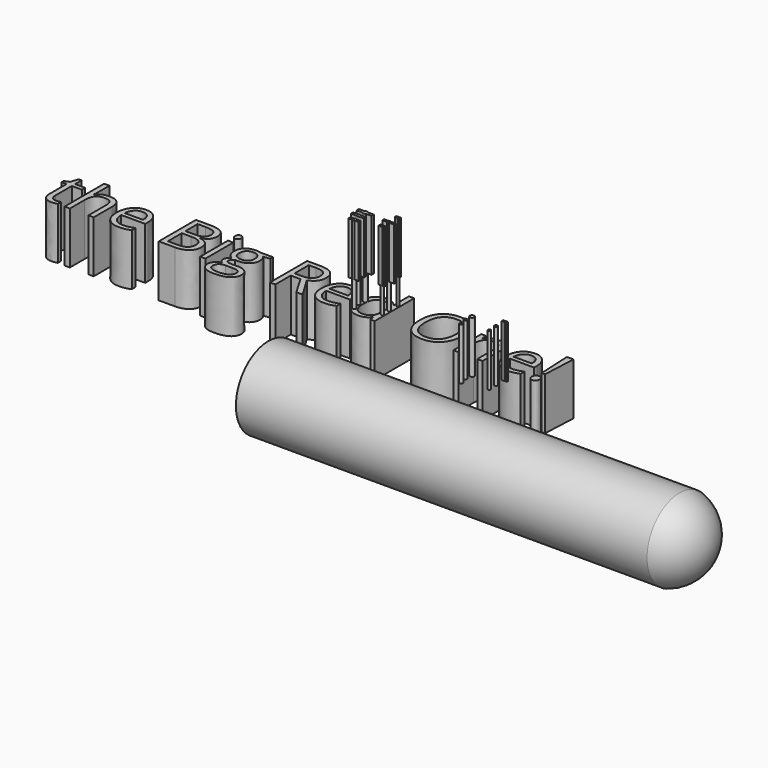
from build123d import *

# Parameters (mm, degrees)
F2_TEXT_SIZE = 31.8179838359
F3_DEPTH     = 25.4
F4_R         = 1.1140946011
F4_R_2       = 0.7578695581
F4_R_3       = 0.853310294
F4_R_4       = 0.5642153701
F4_R_5       = 0.7545312037
F4_R_6       = 0.6707809487
F5_DEPTH     = 12.7
F7_DEPTH     = 25.4
F6_R         = 0.853310294
F6_R_2       = 0.7578695581
F6_R_3       = 1.1140946011
F6_R_4       = 0.6707809487
F6_R_5       = 0.7545312037


# Not quite as in the source:
# - Text() gives the source's letters only with a copy of the font that has no kerning and outlines rounded to 1/6400 em; it was checked with that copy


with BuildPart() as f1:
    # F0 (on Top) → F1 (revolve)
    with BuildSketch(Plane.XY):
        with BuildLine():
            Line((-109.392100472, 19.84375), (-109.392100472, 0))
            Line((-109.392100472, 0), (86.664149528, 0))
            Line((86.664149528, 0), (106.507899528, 0))
            ThreePointArc((106.507899528, 0), (102.3549554862, 12.4198859765), (91.5666861697, 19.84375))
            Line((91.5666861697, 19.84375), (-109.392100472, 19.84375))
        make_face()
    revolve(axis=Axis((96.586024528, 0, 0), (1, 0, 0)))


with BuildPart() as f3:
    # F2 (on Top) → F3 (new body)
    with BuildSketch(Plane.XY):
        with Locations((-246.8578389671, 29.8468321562)):
            Text('the Big Red One!', F2_TEXT_SIZE, font='Open Sans', text_align=(TextAlign.LEFT, TextAlign.BOTTOM))
    extrude(amount=F3_DEPTH)

    # F4 (on face) → F5 (join)
    with BuildSketch(Plane.XY.offset(25.4)):
        with Locations((-94.5394486189, 40.5866801739)):
            Circle(F4_R)
        with Locations((-94.986744225, 37.075035274)):
            Circle(F4_R_2)
        with Locations((-94.0843075514, 33.4260687232)):
            Circle(F4_R_3)
        with Locations((-82.2114273906, 45.2312678099)):
            Circle(F4_R_4)
        with Locations((-82.5017765164, 40.1796028018)):
            Circle(F4_R_5)
        with Locations((-82.3683738708, 35.9273776412)):
            Circle(F4_R_6)
    extrude(amount=F5_DEPTH)

    # F6 (on face) → F7 (join)
    with BuildSketch(Plane.XY.offset(38.1)):
        with BuildLine():
            ThreePointArc((-93.522393393, 32.7838920057), (-93.3072536299, 33.0734702815), (-93.2309972573, 33.4260687232))
            ThreePointArc((-93.2309972573, 33.4260687232), (-93.3072536299, 33.7786671649), (-93.522393393, 34.0682454407))
            Line((-93.522393393, 34.0682454407), (-94.6462217098, 34.0682454407))
            ThreePointArc((-94.6462217098, 34.0682454407), (-94.9376178454, 33.4260687232), (-94.6462217098, 32.7838920057))
            Line((-94.6462217098, 32.7838920057), (-93.522393393, 32.7838920057))
        make_face()
        with BuildLine():
            ThreePointArc((-93.522393393, 34.0682454407), (-93.3072536299, 33.7786671649), (-93.2309972573, 33.4260687232))
            ThreePointArc((-93.2309972573, 33.4260687232), (-93.3072536299, 33.0734702815), (-93.522393393, 32.7838920057))
            Line((-93.522393393, 32.7838920057), (-91.6549861431, 32.7838920057))
            Line((-91.6549861431, 32.7838920057), (-91.6549861431, 34.0682454407))
            Line((-91.6549861431, 34.0682454407), (-93.522393393, 34.0682454407))
        make_face()
        with BuildLine():
            Line((-94.6462217098, 34.0682454407), (-93.522393393, 34.0682454407))
            ThreePointArc((-93.522393393, 34.0682454407), (-94.0843075514, 34.2793790173), (-94.6462217098, 34.0682454407))
        make_face()
        with BuildLine():
            ThreePointArc((-94.6462217098, 32.7838920057), (-94.0843075514, 32.5727584292), (-93.522393393, 32.7838920057))
            Line((-93.522393393, 32.7838920057), (-94.6462217098, 32.7838920057))
        make_face()
        with BuildLine():
            ThreePointArc((-94.6462217098, 32.7838920057), (-94.9376178454, 33.4260687232), (-94.6462217098, 34.0682454407))
            Line((-94.6462217098, 34.0682454407), (-96.5136289597, 34.0682454407))
            Line((-96.5136289597, 34.0682454407), (-96.5136289597, 32.7838920057))
            Line((-96.5136289597, 32.7838920057), (-94.6462217098, 32.7838920057))
        make_face()
        with BuildLine():
            ThreePointArc((-94.6923237196, 36.3766923547), (-94.3552782301, 36.6559684961), (-94.228874667, 37.075035274))
            ThreePointArc((-94.228874667, 37.075035274), (-94.3552782301, 37.4941020519), (-94.6923237196, 37.7733781934))
            Line((-94.6923237196, 37.7733781934), (-95.2811647305, 37.7733781934))
            ThreePointArc((-95.2811647305, 37.7733781934), (-95.7446137831, 37.075035274), (-95.2811647305, 36.3766923547))
            Line((-95.2811647305, 36.3766923547), (-94.6923237196, 36.3766923547))
        make_face()
        with BuildLine():
            ThreePointArc((-94.6923237196, 37.7733781934), (-94.3552782301, 37.4941020519), (-94.228874667, 37.075035274))
            ThreePointArc((-94.228874667, 37.075035274), (-94.3552782301, 36.6559684961), (-94.6923237196, 36.3766923547))
            Line((-94.6923237196, 36.3766923547), (-91.8325185776, 36.3766923547))
            Line((-91.8325185776, 36.3766923547), (-91.8325185776, 37.7733781934))
            Line((-91.8325185776, 37.7733781934), (-94.6923237196, 37.7733781934))
        make_face()
        with BuildLine():
            Line((-95.2811647305, 37.7733781934), (-94.6923237196, 37.7733781934))
            ThreePointArc((-94.6923237196, 37.7733781934), (-94.986744225, 37.8329048321), (-95.2811647305, 37.7733781934))
        make_face()
        with BuildLine():
            ThreePointArc((-95.2811647305, 36.3766923547), (-94.986744225, 36.317165716), (-94.6923237196, 36.3766923547))
            Line((-94.6923237196, 36.3766923547), (-95.2811647305, 36.3766923547))
        make_face()
        with BuildLine():
            ThreePointArc((-95.2811647305, 36.3766923547), (-95.7446137831, 37.075035274), (-95.2811647305, 37.7733781934))
            Line((-95.2811647305, 37.7733781934), (-98.1409698725, 37.7733781934))
            Line((-98.1409698725, 37.7733781934), (-98.1409698725, 36.3766923547))
            Line((-98.1409698725, 36.3766923547), (-95.2811647305, 36.3766923547))
        make_face()
        with BuildLine():
            ThreePointArc((-93.6806709547, 39.8769564927), (-93.4911246376, 40.2095547167), (-93.4253540178, 40.5866801739))
            ThreePointArc((-93.4253540178, 40.5866801739), (-93.4911246376, 40.9638056311), (-93.6806709547, 41.2964038551))
            Line((-93.6806709547, 41.2964038551), (-95.3982262831, 41.2964038551))
            ThreePointArc((-95.3982262831, 41.2964038551), (-95.65354322, 40.5866801739), (-95.3982262831, 39.8769564927))
            Line((-95.3982262831, 39.8769564927), (-93.6806709547, 39.8769564927))
        make_face()
        with BuildLine():
            ThreePointArc((-93.6806709547, 41.2964038551), (-93.4911246376, 40.9638056311), (-93.4253540178, 40.5866801739))
            ThreePointArc((-93.4253540178, 40.5866801739), (-93.4911246376, 40.2095547167), (-93.6806709547, 39.8769564927))
            Line((-93.6806709547, 39.8769564927), (-90.9057930112, 39.8769564927))
            Line((-90.9057930112, 39.8769564927), (-90.9057930112, 41.2964038551))
            Line((-90.9057930112, 41.2964038551), (-93.6806709547, 41.2964038551))
        make_face()
        with BuildLine():
            Line((-95.3982262831, 41.2964038551), (-93.6806709547, 41.2964038551))
            ThreePointArc((-93.6806709547, 41.2964038551), (-94.5394486189, 41.700774775), (-95.3982262831, 41.2964038551))
        make_face()
        with BuildLine():
            ThreePointArc((-95.3982262831, 39.8769564927), (-94.5394486189, 39.4725855728), (-93.6806709547, 39.8769564927))
            Line((-93.6806709547, 39.8769564927), (-95.3982262831, 39.8769564927))
        make_face()
        with BuildLine():
            ThreePointArc((-95.3982262831, 39.8769564927), (-95.65354322, 40.5866801739), (-95.3982262831, 41.2964038551))
            Line((-95.3982262831, 41.2964038551), (-98.1731042266, 41.2964038551))
            Line((-98.1731042266, 41.2964038551), (-98.1731042266, 39.8769564927))
            Line((-98.1731042266, 39.8769564927), (-95.3982262831, 39.8769564927))
        make_face()
        with BuildLine():
            ThreePointArc((-82.0070981772, 35.3621989489), (-81.780035561, 35.6051896304), (-81.6975929222, 35.9273776412))
            ThreePointArc((-81.6975929222, 35.9273776412), (-81.780035561, 36.249565652), (-82.0070981772, 36.4925563335))
            Line((-82.0070981772, 36.4925563335), (-82.7296495645, 36.4925563335))
            ThreePointArc((-82.7296495645, 36.4925563335), (-83.0391548195, 35.9273776412), (-82.7296495645, 35.3621989489))
            Line((-82.7296495645, 35.3621989489), (-82.0070981772, 35.3621989489))
        make_face()
        with BuildLine():
            ThreePointArc((-82.0070981772, 36.4925563335), (-81.780035561, 36.249565652), (-81.6975929222, 35.9273776412))
            ThreePointArc((-81.6975929222, 35.9273776412), (-81.780035561, 35.6051896304), (-82.0070981772, 35.3621989489))
            Line((-82.0070981772, 35.3621989489), (-80.9701830149, 35.3621989489))
            Line((-80.9701830149, 35.3621989489), (-80.9701830149, 36.4925563335))
            Line((-80.9701830149, 36.4925563335), (-82.0070981772, 36.4925563335))
        make_face()
        with BuildLine():
            Line((-82.7296495645, 36.4925563335), (-82.0070981772, 36.4925563335))
            ThreePointArc((-82.0070981772, 36.4925563335), (-82.3683738708, 36.5981585899), (-82.7296495645, 36.4925563335))
        make_face()
        with BuildLine():
            ThreePointArc((-82.7296495645, 35.3621989489), (-82.3683738708, 35.2565966925), (-82.0070981772, 35.3621989489))
            Line((-82.0070981772, 35.3621989489), (-82.7296495645, 35.3621989489))
        make_face()
        with BuildLine():
            ThreePointArc((-82.7296495645, 35.3621989489), (-83.0391548195, 35.9273776412), (-82.7296495645, 36.4925563335))
            Line((-82.7296495645, 36.4925563335), (-83.7665647268, 36.4925563335))
            Line((-83.7665647268, 36.4925563335), (-83.7665647268, 35.3621989489))
            Line((-83.7665647268, 35.3621989489), (-82.7296495645, 35.3621989489))
        make_face()
        with BuildLine():
            ThreePointArc((-82.0221924238, 39.597094059), (-81.8194355093, 39.8575343505), (-81.7472453127, 40.1796028018))
            ThreePointArc((-81.7472453127, 40.1796028018), (-81.8194355093, 40.5016712531), (-82.0221924238, 40.7621115446))
            Line((-82.0221924238, 40.7621115446), (-82.9813606091, 40.7621115446))
            ThreePointArc((-82.9813606091, 40.7621115446), (-83.2563077201, 40.1796028018), (-82.9813606091, 39.597094059))
            Line((-82.9813606091, 39.597094059), (-82.0221924238, 39.597094059))
        make_face()
        with BuildLine():
            ThreePointArc((-82.0221924238, 40.7621115446), (-81.8194355093, 40.5016712531), (-81.7472453127, 40.1796028018))
            ThreePointArc((-81.7472453127, 40.1796028018), (-81.8194355093, 39.8575343505), (-82.0221924238, 39.597094059))
            Line((-82.0221924238, 39.597094059), (-79.5959383249, 39.597094059))
            Line((-79.5959383249, 39.597094059), (-79.5959383249, 40.7621115446))
            Line((-79.5959383249, 40.7621115446), (-82.0221924238, 40.7621115446))
        make_face()
        with BuildLine():
            Line((-82.9813606091, 40.7621115446), (-82.0221924238, 40.7621115446))
            ThreePointArc((-82.0221924238, 40.7621115446), (-82.5017765164, 40.9341340055), (-82.9813606091, 40.7621115446))
        make_face()
        with BuildLine():
            ThreePointArc((-82.9813606091, 39.597094059), (-82.5017765164, 39.4250715981), (-82.0221924238, 39.597094059))
            Line((-82.0221924238, 39.597094059), (-82.9813606091, 39.597094059))
        make_face()
        with BuildLine():
            ThreePointArc((-82.9813606091, 39.597094059), (-83.2563077201, 40.1796028018), (-82.9813606091, 40.7621115446))
            Line((-82.9813606091, 40.7621115446), (-85.4076147079, 40.7621115446))
            Line((-85.4076147079, 40.7621115446), (-85.4076147079, 39.597094059))
            Line((-85.4076147079, 39.597094059), (-82.9813606091, 39.597094059))
        make_face()
        with BuildLine():
            ThreePointArc((-81.8173954273, 44.8274388909), (-81.6914957249, 45.0121558592), (-81.6472120205, 45.2312678099))
            ThreePointArc((-81.6472120205, 45.2312678099), (-81.6914957249, 45.4503797605), (-81.8173954273, 45.6350967288))
            Line((-81.8173954273, 45.6350967288), (-82.6054593539, 45.6350967288))
            ThreePointArc((-82.6054593539, 45.6350967288), (-82.7756427607, 45.2312678099), (-82.6054593539, 44.8274388909))
            Line((-82.6054593539, 44.8274388909), (-81.8173954273, 44.8274388909))
        make_face()
        with BuildLine():
            ThreePointArc((-81.8173954273, 45.6350967288), (-81.6914957249, 45.4503797605), (-81.6472120205, 45.2312678099))
            ThreePointArc((-81.6472120205, 45.2312678099), (-81.6914957249, 45.0121558592), (-81.8173954273, 44.8274388909))
            Line((-81.8173954273, 44.8274388909), (-80.9738710523, 44.8274388909))
            Line((-80.9738710523, 44.8274388909), (-80.9738710523, 45.6350967288))
            Line((-80.9738710523, 45.6350967288), (-81.8173954273, 45.6350967288))
        make_face()
        with BuildLine():
            Line((-82.6054593539, 45.6350967288), (-81.8173954273, 45.6350967288))
            ThreePointArc((-81.8173954273, 45.6350967288), (-82.2114273906, 45.79548318), (-82.6054593539, 45.6350967288))
        make_face()
        with BuildLine():
            ThreePointArc((-82.6054593539, 44.8274388909), (-82.2114273906, 44.6670524398), (-81.8173954273, 44.8274388909))
            Line((-81.8173954273, 44.8274388909), (-82.6054593539, 44.8274388909))
        make_face()
        with BuildLine():
            ThreePointArc((-82.6054593539, 44.8274388909), (-82.7756427607, 45.2312678099), (-82.6054593539, 45.6350967288))
            Line((-82.6054593539, 45.6350967288), (-83.4489837289, 45.6350967288))
            Line((-83.4489837289, 45.6350967288), (-83.4489837289, 44.8274388909))
            Line((-83.4489837289, 44.8274388909), (-82.6054593539, 44.8274388909))
        make_face()
    extrude(amount=F7_DEPTH)


with BuildPart() as f7:
    # F6 (on face) → F7, piece 2 (new body)
    with BuildSketch(Plane.XY.offset(38.1)):
        with Locations((-8.4707425399, -8.2632377744)):
            Circle(F6_R)
    extrude(amount=F7_DEPTH)


with BuildPart() as f7b:
    # F6 (on face) → F7, piece 3 (new body)
    with BuildSketch(Plane.XY.offset(38.1)):
        with Locations((-9.3731792136, -4.6142712235)):
            Circle(F6_R_2)
    extrude(amount=F7_DEPTH)


with BuildPart() as f7c:
    # F6 (on face) → F7, piece 4 (new body)
    with BuildSketch(Plane.XY.offset(38.1)):
        with Locations((-8.9258836074, -1.1026263237)):
            Circle(F6_R_3)
    extrude(amount=F7_DEPTH)


with BuildPart() as f7d:
    # F6 (on face) → F7, piece 5 (new body)
    with BuildSketch(Plane.XY.offset(38.1)):
        with Locations((3.2451911406, -5.7619288564)):
            Circle(F6_R_4)
    extrude(amount=F7_DEPTH)


with BuildPart() as f7e:
    # F6 (on face) → F7, piece 6 (new body)
    with BuildSketch(Plane.XY.offset(38.1)):
        with Locations((3.111788495, -1.5097036958)):
            Circle(F6_R_5)
    extrude(amount=F7_DEPTH)


with BuildPart() as f7f:
    # F6 (on face) → F7, piece 7 (new body)
    with BuildSketch(Plane.XY.offset(38.1)):
        with BuildLine():
            ThreePointArc((3.7961695842, 3.1381323934), (3.9220692865, 3.3228493616), (3.966352991, 3.5419613123))
            ThreePointArc((3.966352991, 3.5419613123), (3.9220692865, 3.761073263), (3.7961695842, 3.9457902312))
            Line((3.7961695842, 3.9457902312), (3.0081056576, 3.9457902312))
            ThreePointArc((3.0081056576, 3.9457902312), (2.8379222508, 3.5419613123), (3.0081056576, 3.1381323934))
            Line((3.0081056576, 3.1381323934), (3.7961695842, 3.1381323934))
        make_face()
        with BuildLine():
            ThreePointArc((3.7961695842, 3.9457902312), (3.9220692865, 3.761073263), (3.966352991, 3.5419613123))
            ThreePointArc((3.966352991, 3.5419613123), (3.9220692865, 3.3228493616), (3.7961695842, 3.1381323934))
            Line((3.7961695842, 3.1381323934), (4.6396939592, 3.1381323934))
            Line((4.6396939592, 3.1381323934), (4.6396939592, 3.9457902312))
            Line((4.6396939592, 3.9457902312), (3.7961695842, 3.9457902312))
        make_face()
        with BuildLine():
            Line((3.0081056576, 3.9457902312), (3.7961695842, 3.9457902312))
            ThreePointArc((3.7961695842, 3.9457902312), (3.4021376209, 4.1061766824), (3.0081056576, 3.9457902312))
        make_face()
        with BuildLine():
            ThreePointArc((3.0081056576, 3.1381323934), (3.4021376209, 2.9777459422), (3.7961695842, 3.1381323934))
            Line((3.7961695842, 3.1381323934), (3.0081056576, 3.1381323934))
        make_face()
        with BuildLine():
            ThreePointArc((3.0081056576, 3.1381323934), (2.8379222508, 3.5419613123), (3.0081056576, 3.9457902312))
            Line((3.0081056576, 3.9457902312), (2.1645812826, 3.9457902312))
            Line((2.1645812826, 3.9457902312), (2.1645812826, 3.1381323934))
            Line((2.1645812826, 3.1381323934), (3.0081056576, 3.1381323934))
        make_face()
    extrude(amount=F7_DEPTH)


solid = Compound([f1.part, f3.part, f7.part, f7b.part, f7c.part, f7d.part, f7e.part, f7f.part])
